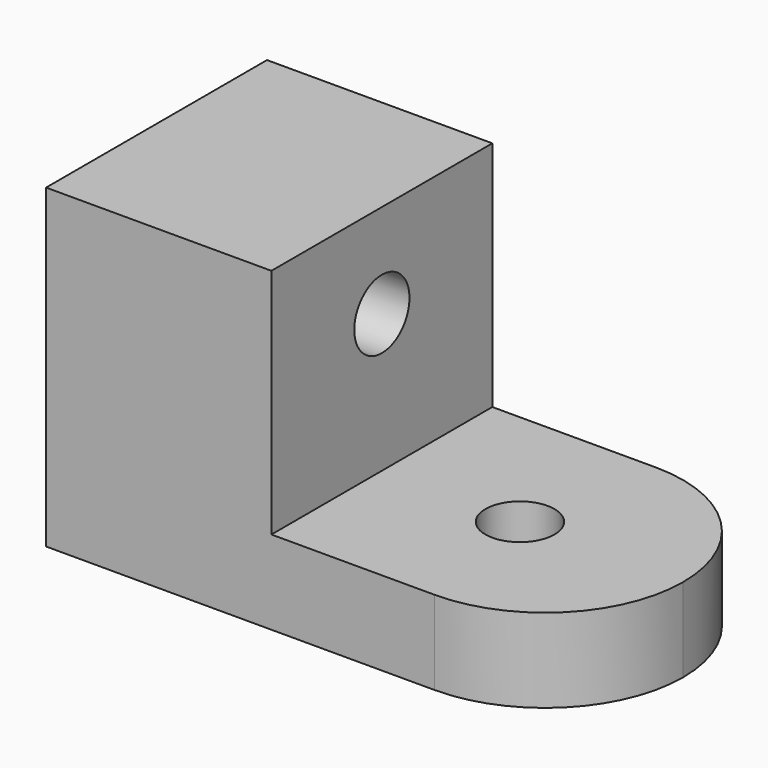
from build123d import *

# Parameters (mm, degrees)
F1_DEPTH = 12.7
F2_R     = 12.69999
F4_D     = 6.35
F6_D     = 6.35


# Not quite as in the source:
# - a fillet or chamfer is up to 0.001 mm smaller than in the source, because OpenCascade refuses the exact size


with BuildPart() as f1:
    # F0 (on Front) → F1 (new body, symmetric)
    with BuildSketch(Plane.XZ):
        Polygon((27.7143083513, 0), (0, 0), (0, 21.3540010154), (-20.7254812121, 21.3540010154), (-20.7254812121, -7.7118072659), (27.7143083513, -7.7118072659), align=None)
    extrude(amount=F1_DEPTH, both=True)

    # F2 (radius 12.7 in the source; OpenCascade refuses exactly that, so slightly less here)
    f2_edges = [f1.edges().sort_by_distance(p)[0] for p in [
        (27.714308, -12.7, -3.855904),
        (27.714308, 12.7, -3.855904),
    ]]
    fillet(f2_edges, radius=F2_R)

    # F4 (through all)
    with Locations(Plane.XY):
        with Locations((12.7, 0)):
            Hole(F4_D / 2)

    # F6 (through all)
    with Locations(Plane.YZ):
        with Locations((0, 12.7)):
            Hole(F6_D / 2)


solid = f1.part
